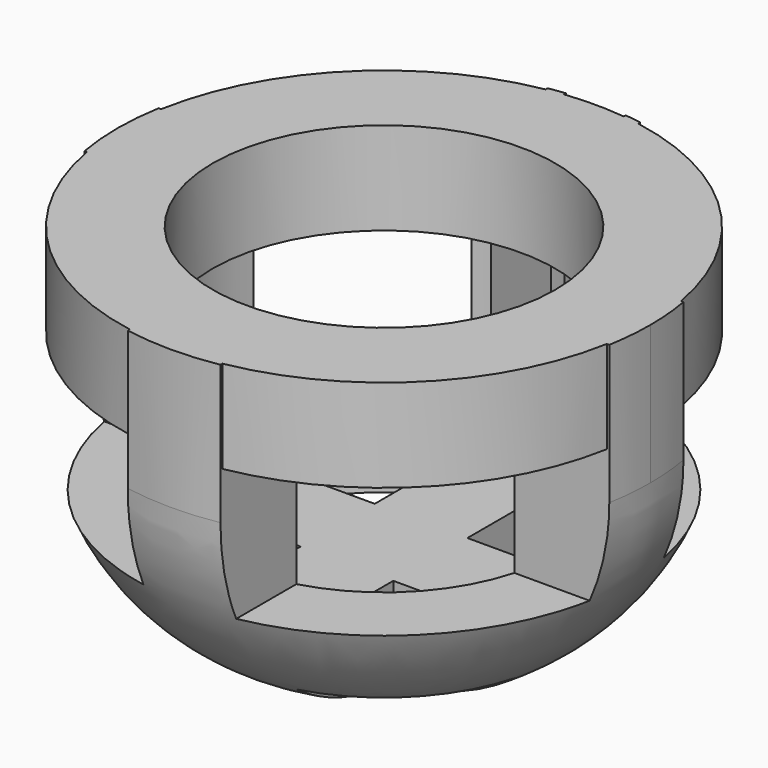
from build123d import *

# Parameters (mm, degrees)
F1_DEPTH = 3
F2_DEPTH = 8
F0_W     = 2
F0_H     = 2
F3_DEPTH = 2
F4_R     = 3.6974991887
F5_DEPTH = 2


# Not quite as in the source:
# - a fillet or chamfer that OpenCascade refuses, or shapes differently, is made with other operations: its cross-section is extruded or revolved along the edge and cut away or added


with BuildPart() as f1:
    # F0 (on Top) → F1 (new body)
    with BuildSketch(Plane.XY):
        with BuildLine():
            Line((3.7669987963, -1), (3.6142080737, -1))
            ThreePointArc((3.6142080737, -1), (2.6516504294, -2.6516504294), (1, -3.6142080737))
            Line((1, -3.6142080737), (1, -5.6623758265))
            ThreePointArc((1, -5.6623758265), (4.0658639918, -4.0658639918), (5.6623758265, -1))
            Line((5.6623758265, -1), (3.7669987963, -1))
        make_face()
    extrude(amount=F1_DEPTH)



with BuildPart() as f1b:
    # F0 (on Top) → F1, piece 2 (new body)
    with BuildSketch(Plane.XY):
        with BuildLine():
            Line((-1, -5.6623758265), (-1, -3.6142080737))
            ThreePointArc((-1, -3.6142080737), (-2.6516504294, -2.6516504294), (-3.6142080737, -1))
            Line((-3.6142080737, -1), (-5.6623758265, -1))
            ThreePointArc((-5.6623758265, -1), (-4.0658639918, -4.0658639918), (-1, -5.6623758265))
        make_face()
    extrude(amount=F1_DEPTH)


with BuildPart() as f1c:
    # F0 (on Top) → F1, piece 3 (new body)
    with BuildSketch(Plane.XY):
        with BuildLine():
            ThreePointArc((-3.6142080737, 1), (-2.6516504294, 2.6516504294), (-1, 3.6142080737))
            Line((-1, 3.6142080737), (-1, 5.6623758265))
            ThreePointArc((-1, 5.6623758265), (-4.0658639918, 4.0658639918), (-5.6623758265, 1))
            Line((-5.6623758265, 1), (-3.6142080737, 1))
        make_face()
    extrude(amount=F1_DEPTH)


with BuildPart() as f1d:
    # F0 (on Top) → F1, piece 4 (new body)
    with BuildSketch(Plane.XY):
        with BuildLine():
            ThreePointArc((1, 3.6142080737), (2.6516504294, 2.6516504294), (3.6142080737, 1))
            Line((3.6142080737, 1), (5.6623758265, 1))
            ThreePointArc((5.6623758265, 1), (4.0658639918, 4.0658639918), (1, 5.6623758265))
            Line((1, 5.6623758265), (1, 3.6142080737))
        make_face()
    extrude(amount=F1_DEPTH)


with BuildPart() as f1_1:
    add(f1.part)

    add(f1b.part)  # F2 merges F1b

    add(f1c.part)  # F2 merges F1c

    add(f1d.part)  # F2 merges F1d
    # F0 (on Top) → F2 (join)
    with BuildSketch(Plane.XY):
        with BuildLine():
            ThreePointArc((0.6450651563, 3.6941021838), (0.8235020396, 3.6584620253), (1, 3.6142080737))
            Line((1, 3.6142080737), (1, 5.6623758265))
            ThreePointArc((1, 5.6623758265), (0.8229328266, 5.6908067585), (0.6450651563, 5.7137020349))
            Line((0.6450651563, 5.7137020349), (0.6450651563, 3.6941021838))
        make_face()
        with BuildLine():
            ThreePointArc((-1, 3.6142080737), (-0.8235020396, 3.6584620253), (-0.6450651563, 3.6941021838))
            Line((-0.6450651563, 3.6941021838), (-0.6450651563, 5.7137020349))
            ThreePointArc((-0.6450651563, 5.7137020349), (-0.8229328266, 5.6908067585), (-1, 5.6623758265))
            Line((-1, 5.6623758265), (-1, 3.6142080737))
        make_face()
        with BuildLine():
            ThreePointArc((-3.6142080737, -1), (-3.75, 0), (-3.6142080737, 1))
            Line((-3.6142080737, 1), (-5.6623758265, 1))
            ThreePointArc((-5.6623758265, 1), (-5.75, 0), (-5.6623758265, -1))
            Line((-5.6623758265, -1), (-3.6142080737, -1))
        make_face()
        with BuildLine():
            ThreePointArc((3.6142080737, 1), (3.7158969493, 0.5045888047), (3.75, 0))
            ThreePointArc((3.75, 0), (3.7158969493, -0.5045888047), (3.6142080737, -1))
            Line((3.6142080737, -1), (3.7669987963, -1))
            Line((3.7669987963, -1), (5.6623758265, -1))
            ThreePointArc((5.6623758265, -1), (5.7280520686, -0.5019158285), (5.75, 0))
            ThreePointArc((5.75, 0), (5.7280520686, 0.5019158285), (5.6623758265, 1))
            Line((5.6623758265, 1), (3.6142080737, 1))
        make_face()
        with BuildLine():
            Line((1, -5.6623758265), (1, -3.6142080737))
            ThreePointArc((1, -3.6142080737), (0, -3.75), (-1, -3.6142080737))
            Line((-1, -3.6142080737), (-1, -5.6623758265))
            ThreePointArc((-1, -5.6623758265), (0, -5.75), (1, -5.6623758265))
        make_face()
    extrude(amount=F2_DEPTH)

    # F0 (on Top) → F3 (join)
    with BuildSketch(Plane.XY):
        with BuildLine():
            ThreePointArc((-0.6450651563, 3.6941021838), (0, 3.75), (0.6450651563, 3.6941021838))
            Line((0.6450651563, 3.6941021838), (0.6450651563, 5.7137020349))
            ThreePointArc((0.6450651563, 5.7137020349), (0, 5.75), (-0.6450651563, 5.7137020349))
            Line((-0.6450651563, 5.7137020349), (-0.6450651563, 3.6941021838))
        make_face()
        with BuildLine():
            Line((0.6450651563, 3.1745089218), (0.6450651563, 3.6941021838))
            ThreePointArc((0.6450651563, 3.6941021838), (0, 3.75), (-0.6450651563, 3.6941021838))
            Line((-0.6450651563, 3.6941021838), (-0.6450651563, 3.1745089218))
            Line((-0.6450651563, 3.1745089218), (0.6450651563, 3.1745089218))
        make_face()
        with BuildLine():
            Line((1, 1), (1, 3.6142080737))
            ThreePointArc((1, 3.6142080737), (0.8235020396, 3.6584620253), (0.6450651563, 3.6941021838))
            Line((0.6450651563, 3.6941021838), (0.6450651563, 3.1745089218))
            Line((0.6450651563, 3.1745089218), (-0.6450651563, 3.1745089218))
            Line((-0.6450651563, 3.1745089218), (-0.6450651563, 3.6941021838))
            ThreePointArc((-0.6450651563, 3.6941021838), (-0.8235020396, 3.6584620253), (-1, 3.6142080737))
            Line((-1, 3.6142080737), (-1, 1))
            Line((-1, 1), (1, 1))
        make_face()
        with BuildLine():
            Line((-1, -1), (-1, 1))
            Line((-1, 1), (-3.6142080737, 1))
            ThreePointArc((-3.6142080737, 1), (-3.75, 0), (-3.6142080737, -1))
            Line((-3.6142080737, -1), (-1, -1))
        make_face()
        with BuildLine():
            ThreePointArc((3.6142080737, -1), (3.7158969493, -0.5045888047), (3.75, 0))
            ThreePointArc((3.75, 0), (3.7158969493, 0.5045888047), (3.6142080737, 1))
            Line((3.6142080737, 1), (1, 1))
            Line((1, 1), (1, -1))
            Line((1, -1), (3.6142080737, -1))
        make_face()
        Rectangle(F0_W, F0_H)
        with BuildLine():
            ThreePointArc((-1, -3.6142080737), (0, -3.75), (1, -3.6142080737))
            Line((1, -3.6142080737), (1, -1))
            Line((1, -1), (-1, -1))
            Line((-1, -1), (-1, -3.6142080737))
        make_face()
    extrude(amount=F3_DEPTH)

    # F4 (on face) → F5 (join)
    with BuildSketch(Plane.XY.offset(8)):
        with BuildLine():
            Line((3.6142080737, 1), (5.609054912, 1))
            ThreePointArc((5.609054912, 1), (-5.6974991887, 0), (5.609054912, -1))
            Line((5.609054912, -1), (3.6142080737, -1))
            ThreePointArc((3.6142080737, -1), (3.75, 0), (3.6142080737, 1))
        make_face()
        Circle(F4_R, mode=Mode.SUBTRACT)
    extrude(amount=-F5_DEPTH)

    # F6: fillet of radius 5 on 1 edges, made by hand

    # F6_s1 → F6_t2 (revolve, cut)
    with BuildSketch(Plane(origin=(0, 0, 0), x_dir=(0, 0, 1), z_dir=(-0.1739130435, 0.9847610133, 0))):
        with BuildLine():
            ThreePointArc((0, 0.75), (1.4644660941, 4.2855339059), (5, 5.75))
            Line((5, 5.75), (0, 5.75))
            Line((0, 5.75), (0, 0.75))
        make_face()
    revolve(axis=Axis((0, 0, 0), (0, 0, -1)), mode=Mode.SUBTRACT)


solid = f1_1.part
